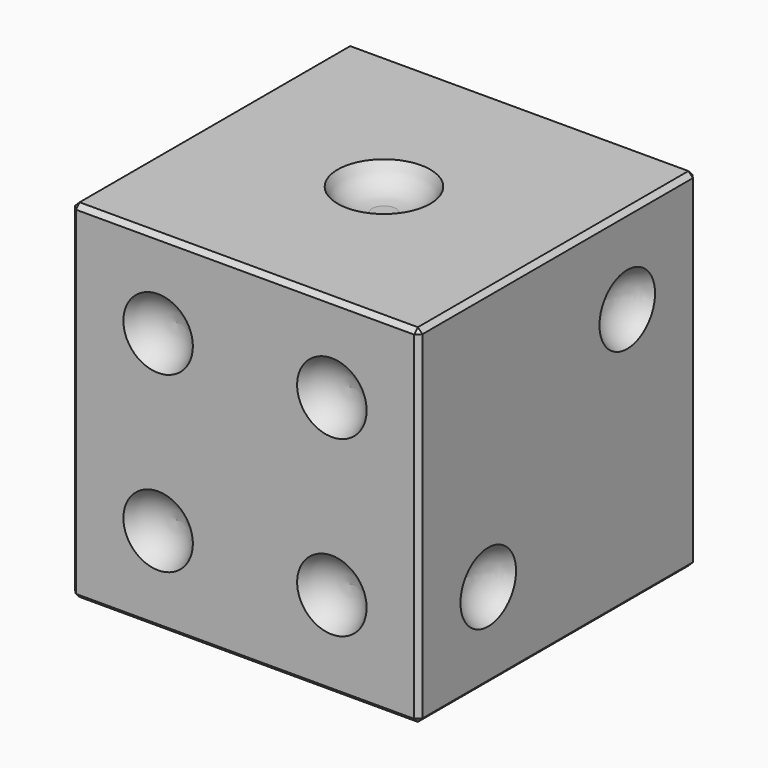
from build123d import *

# Parameters (mm, degrees)
F0_W      = 15
F0_H      = 15
F1_DEPTH  = 15
F2_R      = 2
F3_DEPTH  = 1
F4_R      = 1.5
F5_DEPTH  = 1
F6_R      = 1.5
F7_DEPTH  = 1
F8_R      = 1.5
F9_DEPTH  = 1
F10_R     = 1.5
F11_DEPTH = 1
F12_R     = 1.5
F13_DEPTH = 1
F15_SIZE  = 0.2


# Not quite as in the source:
# - a fillet or chamfer that OpenCascade refuses, or shapes differently, is made with other operations: its cross-section is extruded or revolved along the edge and cut away or added


with BuildPart() as f1:
    # F0 (on Top) → F1 (new body)
    with BuildSketch(Plane.XY):
        with Locations((7.5, 7.5)):
            Rectangle(F0_W, F0_H)
    extrude(amount=F1_DEPTH)

    # F2 (on face) → F3 (cut)
    with BuildSketch(Plane.XY.offset(15)):
        with Locations((7.5, 7.5)):
            Circle(F2_R)
    extrude(amount=-F3_DEPTH, mode=Mode.SUBTRACT)

    # F4 (on face) → F5 (cut)
    with BuildSketch(Plane(origin=(0, 0, 0), x_dir=(1, 0, 0), z_dir=(0, 0, -1))):
        with Locations((5, -3.75)):
            Circle(F4_R)
        with Locations((10, -3.75)):
            Circle(F4_R)
        with Locations((10, -7.5)):
            Circle(F4_R)
        with Locations((5, -7.5)):
            Circle(F4_R)
        with Locations((5, -11.25)):
            Circle(F4_R)
        with Locations((10, -11.25)):
            Circle(F4_R)
    extrude(amount=-F5_DEPTH, mode=Mode.SUBTRACT)

    # F6 (on face) → F7 (cut)
    with BuildSketch(Plane.YZ.offset(15)):
        with Locations((3.75, 3.75)):
            Circle(F6_R)
        with Locations((11.25, 11.25)):
            Circle(F6_R)
    extrude(amount=-F7_DEPTH, mode=Mode.SUBTRACT)

    # F8 (on face) → F9 (cut)
    with BuildSketch(Plane(origin=(0, 0, 0), x_dir=(0, -1, 0), z_dir=(-1, 0, 0))):
        with Locations((-11.25, 11.25)):
            Circle(F8_R)
        with Locations((-7.5, 7.5)):
            Circle(F8_R)
        with Locations((-11.25, 3.75)):
            Circle(F8_R)
        with Locations((-3.75, 3.75)):
            Circle(F8_R)
        with Locations((-3.75, 11.25)):
            Circle(F8_R)
    extrude(amount=-F9_DEPTH, mode=Mode.SUBTRACT)

    # F10 (on face) → F11 (cut)
    with BuildSketch(Plane(origin=(0, 15, 0), x_dir=(-1, 0, 0), z_dir=(0, 1, 0))):
        with Locations((-3.75, 11.25)):
            Circle(F10_R)
        with Locations((-7.5, 7.5)):
            Circle(F10_R)
        with Locations((-11.25, 3.75)):
            Circle(F10_R)
    extrude(amount=-F11_DEPTH, mode=Mode.SUBTRACT)

    # F12 (on face) → F13 (cut)
    with BuildSketch(Plane.XZ):
        with Locations((3.75, 11.25)):
            Circle(F12_R)
        with Locations((11.25, 11.25)):
            Circle(F12_R)
        with Locations((11.25, 3.75)):
            Circle(F12_R)
        with Locations((3.75, 3.75)):
            Circle(F12_R)
    extrude(amount=-F13_DEPTH, mode=Mode.SUBTRACT)

    # F14: fillet of radius 1.6 on 21 edges, made by hand

    # F14_s1 → F14_t2 (revolve)
    with BuildSketch(Plane.XY.offset(3.75)):
        with BuildLine():
            ThreePointArc((0, 9.75), (0.7266499161, 10.3388125064), (1, 11.2332396974))
            Line((1, 11.2332396974), (1, 9.75))
            Line((1, 9.75), (0, 9.75))
        make_face()
    revolve(axis=Axis((1, 11.25, 3.75), (-1, 0, 0)))

    # F14_s3 → F14_t4 (revolve)
    with BuildSketch(Plane.XY.offset(7.5)):
        with BuildLine():
            ThreePointArc((0, 6), (0.7266499161, 6.5888125064), (1, 7.4832396974))
            Line((1, 7.4832396974), (1, 6))
            Line((1, 6), (0, 6))
        make_face()
    revolve(axis=Axis((1, 7.5, 7.5), (-1, 0, 0)))

    # F14_s5 → F14_t6 (revolve)
    with BuildSketch(Plane.XY.offset(11.25)):
        with BuildLine():
            ThreePointArc((0, 9.75), (0.7266499161, 10.3388125064), (1, 11.2332396974))
            Line((1, 11.2332396974), (1, 9.75))
            Line((1, 9.75), (0, 9.75))
        make_face()
    revolve(axis=Axis((1, 11.25, 11.25), (-1, 0, 0)))

    # F14_s7 → F14_t8 (revolve)
    with BuildSketch(Plane.XY.offset(3.75)):
        with BuildLine():
            ThreePointArc((0, 2.25), (0.7266499161, 2.8388125064), (1, 3.7332396974))
            Line((1, 3.7332396974), (1, 2.25))
            Line((1, 2.25), (0, 2.25))
        make_face()
    revolve(axis=Axis((1, 3.75, 3.75), (-1, 0, 0)))

    # F14_s9 → F14_t10 (revolve)
    with BuildSketch(Plane.XY.offset(11.25)):
        with BuildLine():
            ThreePointArc((0, 2.25), (0.7266499161, 2.8388125064), (1, 3.7332396974))
            Line((1, 3.7332396974), (1, 2.25))
            Line((1, 2.25), (0, 2.25))
        make_face()
    revolve(axis=Axis((1, 3.75, 11.25), (-1, 0, 0)))

    # F14_s11 → F14_t12 (revolve)
    with BuildSketch(Plane.XY.offset(11.25)):
        with BuildLine():
            ThreePointArc((2.25, 15), (2.8388125064, 14.2733500839), (3.7332396974, 14))
            Line((3.7332396974, 14), (2.25, 14))
            Line((2.25, 14), (2.25, 15))
        make_face()
    revolve(axis=Axis((3.75, 14, 11.25), (0, 1, 0)))

    # F14_s13 → F14_t14 (revolve)
    with BuildSketch(Plane.XY.offset(7.5)):
        with BuildLine():
            ThreePointArc((6, 15), (6.5888125064, 14.2733500839), (7.4832396974, 14))
            Line((7.4832396974, 14), (6, 14))
            Line((6, 14), (6, 15))
        make_face()
    revolve(axis=Axis((7.5, 14, 7.5), (0, 1, 0)))

    # F14_s15 → F14_t16 (revolve)
    with BuildSketch(Plane.XY.offset(3.75)):
        with BuildLine():
            ThreePointArc((9.75, 15), (10.3388125064, 14.2733500839), (11.2332396974, 14))
            Line((11.2332396974, 14), (9.75, 14))
            Line((9.75, 14), (9.75, 15))
        make_face()
    revolve(axis=Axis((11.25, 14, 3.75), (0, 1, 0)))

    # F14_s17 → F14_t18 (revolve)
    with BuildSketch(Plane.XZ.offset(-11.25)):
        with BuildLine():
            ThreePointArc((11.5, 0), (10.9111874936, 0.7266499161), (10.0167603026, 1))
            Line((10.0167603026, 1), (11.5, 1))
            Line((11.5, 1), (11.5, 0))
        make_face()
    revolve(axis=Axis((10, 11.25, 1), (0, 0, -1)))

    # F14_s19 → F14_t20 (revolve)
    with BuildSketch(Plane.XZ.offset(-7.5)):
        with BuildLine():
            ThreePointArc((11.5, 0), (10.9111874936, 0.7266499161), (10.0167603026, 1))
            Line((10.0167603026, 1), (11.5, 1))
            Line((11.5, 1), (11.5, 0))
        make_face()
    revolve(axis=Axis((10, 7.5, 1), (0, 0, -1)))

    # F14_s21 → F14_t22 (revolve)
    with BuildSketch(Plane.XZ.offset(-11.25)):
        with BuildLine():
            ThreePointArc((6.5, 0), (5.9111874936, 0.7266499161), (5.0167603026, 1))
            Line((5.0167603026, 1), (6.5, 1))
            Line((6.5, 1), (6.5, 0))
        make_face()
    revolve(axis=Axis((5, 11.25, 1), (0, 0, -1)))

    # F14_s23 → F14_t24 (revolve)
    with BuildSketch(Plane.XZ.offset(-7.5)):
        with BuildLine():
            ThreePointArc((6.5, 0), (5.9111874936, 0.7266499161), (5.0167603026, 1))
            Line((5.0167603026, 1), (6.5, 1))
            Line((6.5, 1), (6.5, 0))
        make_face()
    revolve(axis=Axis((5, 7.5, 1), (0, 0, -1)))

    # F14_s25 → F14_t26 (revolve)
    with BuildSketch(Plane.XZ.offset(-3.75)):
        with BuildLine():
            ThreePointArc((6.5, 0), (5.9111874936, 0.7266499161), (5.0167603026, 1))
            Line((5.0167603026, 1), (6.5, 1))
            Line((6.5, 1), (6.5, 0))
        make_face()
    revolve(axis=Axis((5, 3.75, 1), (0, 0, -1)))

    # F14_s27 → F14_t28 (revolve)
    with BuildSketch(Plane.XZ.offset(-3.75)):
        with BuildLine():
            ThreePointArc((11.5, 0), (10.9111874936, 0.7266499161), (10.0167603026, 1))
            Line((10.0167603026, 1), (11.5, 1))
            Line((11.5, 1), (11.5, 0))
        make_face()
    revolve(axis=Axis((10, 3.75, 1), (0, 0, -1)))

    # F14_s29 → F14_t30 (revolve)
    with BuildSketch(Plane.XY.offset(3.75)):
        with BuildLine():
            ThreePointArc((15, 5.25), (14.2733500839, 4.6611874936), (14, 3.7667603026))
            Line((14, 3.7667603026), (14, 5.25))
            Line((14, 5.25), (15, 5.25))
        make_face()
    revolve(axis=Axis((14, 3.75, 3.75), (1, 0, 0)))

    # F14_s31 → F14_t32 (revolve)
    with BuildSketch(Plane.XY.offset(11.25)):
        with BuildLine():
            ThreePointArc((15, 12.75), (14.2733500839, 12.1611874936), (14, 11.2667603026))
            Line((14, 11.2667603026), (14, 12.75))
            Line((14, 12.75), (15, 12.75))
        make_face()
    revolve(axis=Axis((14, 11.25, 11.25), (1, 0, 0)))

    # F14_s33 → F14_t34 (revolve)
    with BuildSketch(Plane.XZ.offset(-7.5)):
        with BuildLine():
            ThreePointArc((9.5, 15), (8.9111874936, 14.2733500839), (8.0167603026, 14))
            Line((8.0167603026, 14), (9.5, 14))
            Line((9.5, 14), (9.5, 15))
        make_face()
    revolve(axis=Axis((7.5, 7.5, 14), (0, 0, 1)))

    # F14_s35 → F14_t36 (revolve)
    with BuildSketch(Plane.XY.offset(11.25)):
        with BuildLine():
            ThreePointArc((5.25, 0), (4.6611874936, 0.7266499161), (3.7667603026, 1))
            Line((3.7667603026, 1), (5.25, 1))
            Line((5.25, 1), (5.25, 0))
        make_face()
    revolve(axis=Axis((3.75, 1, 11.25), (0, -1, 0)))

    # F14_s37 → F14_t38 (revolve)
    with BuildSketch(Plane.XY.offset(11.25)):
        with BuildLine():
            ThreePointArc((12.75, 0), (12.1611874936, 0.7266499161), (11.2667603026, 1))
            Line((11.2667603026, 1), (12.75, 1))
            Line((12.75, 1), (12.75, 0))
        make_face()
    revolve(axis=Axis((11.25, 1, 11.25), (0, -1, 0)))

    # F14_s39 → F14_t40 (revolve)
    with BuildSketch(Plane.XY.offset(3.75)):
        with BuildLine():
            ThreePointArc((12.75, 0), (12.1611874936, 0.7266499161), (11.2667603026, 1))
            Line((11.2667603026, 1), (12.75, 1))
            Line((12.75, 1), (12.75, 0))
        make_face()
    revolve(axis=Axis((11.25, 1, 3.75), (0, -1, 0)))

    # F14_s41 → F14_t42 (revolve)
    with BuildSketch(Plane.XY.offset(3.75)):
        with BuildLine():
            ThreePointArc((5.25, 0), (4.6611874936, 0.7266499161), (3.7667603026, 1))
            Line((3.7667603026, 1), (5.25, 1))
            Line((5.25, 1), (5.25, 0))
        make_face()
    revolve(axis=Axis((3.75, 1, 3.75), (0, -1, 0)))

    # F15
    f15_edges = [f1.edges().sort_by_distance(p)[0] for p in [
        (15, 0, 7.5),
        (7.5, 0, 0),
        (15, 7.5, 0),
        (0, 7.5, 0),
        (0, 0, 7.5),
        (0, 15, 7.5),
        (7.5, 15, 0),
        (7.5, 15, 15),
        (0, 7.5, 15),
        (7.5, 0, 15),
        (15, 7.5, 15),
        (15, 15, 7.5),
    ]]
    chamfer(f15_edges, length=F15_SIZE)


solid = f1.part
